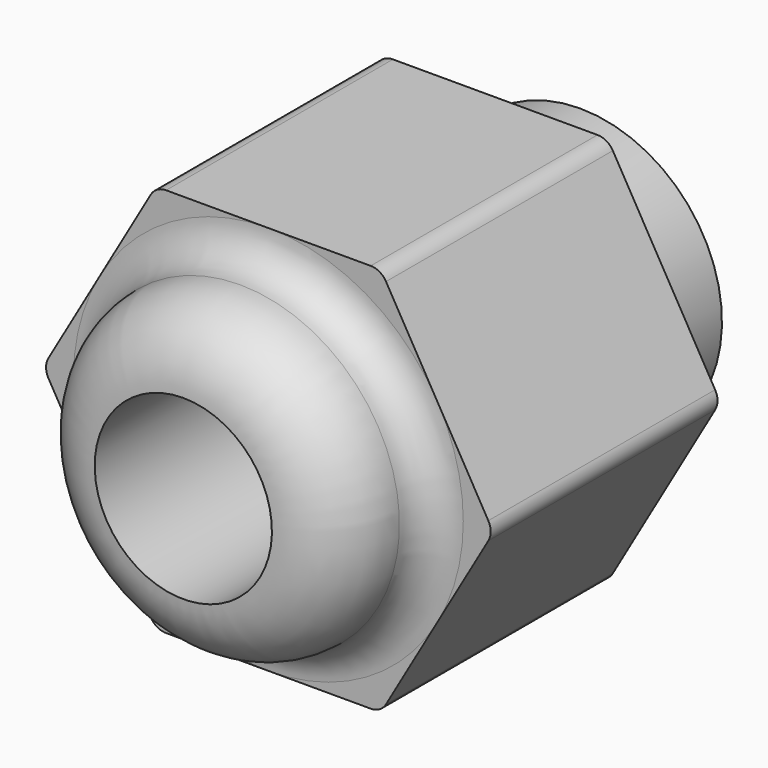
from build123d import *

# Parameters (mm, degrees)
F0_R     = 5
F3_DEPTH = 16
F4_R     = 1.99999
F5_R     = 1


# Not quite as in the source:
# - a fillet or chamfer is up to 0.001 mm smaller than in the source, because OpenCascade refuses the exact size


with BuildPart() as f2:
    # F1 (on Right) → F2 (revolve)
    with BuildSketch(Plane.YZ):
        with BuildLine():
            Line((0, 8), (0, 9))
            Line((0, 9), (-18, 9))
            ThreePointArc((-18, 9), (-20.8284271247, 7.8284271247), (-22, 5))
            Line((-22, 5), (0, 5))
            Line((0, 5), (6, 5))
            Line((6, 5), (6, 8))
            Line((6, 8), (0, 8))
        make_face()
    revolve(axis=Axis((0, -24.3240110576, 0), (0, -1, 0)))

    # F0 (on Front) → F3 (join)
    with BuildSketch(Plane.XZ):
        Polygon((6.3508529611, 11), (-6.3508529611, 11), (-12.7017059222, 0), (-6.3508529611, -11), (6.3508529611, -11), (12.7017059222, 0), align=None)
        Circle(F0_R, mode=Mode.SUBTRACT)
    extrude(amount=F3_DEPTH)

    # F4 (radius 2 in the source; OpenCascade refuses exactly that, so slightly less here)
    f4_edges = [f2.edges().sort_by_distance(p)[0] for p in [
        (0, -16, -9),
    ]]
    fillet(f4_edges, radius=F4_R)

    # F5
    f5_edges = [f2.edges().sort_by_distance(p)[0] for p in [
        (-6.350853, -8, 11),
        (-12.701706, -8, 0),
        (-6.350853, -8, -11),
        (6.350853, -8, -11),
        (12.701706, -8, 0),
        (6.350853, -8, 11),
    ]]
    fillet(f5_edges, radius=F5_R)


solid = f2.part
